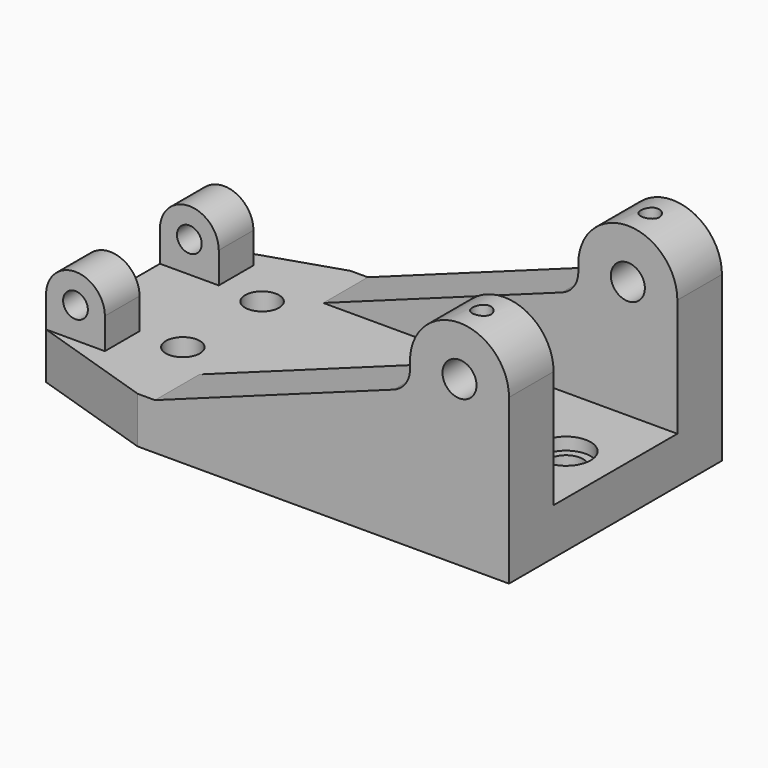
from build123d import *

# Parameters (mm, degrees)
F0_W            = 160
F0_H            = 86
F1_DEPTH        = 15
F3_DEPTH        = 18
F4_R            = 8
F6_D            = 11
F9_DEPTH        = 14
F11_D           = 8
F12_C1_SIZE2    = 13
F12_C1_SIZE     = 40
F12_C2_SIZE2    = 40
F12_C2_SIZE     = 13
F16_D           = 6
F16_DEPTH       = 12
F16_START       = 0.2837665
F16_TIP         = 1.8025818571
F18_D           = 11
F20_D           = 11
F20_CBORE_D     = 16
F20_CBORE_DEPTH = 4


# Not quite as in the source:
# - two fillets or chamfers of one size are made in one step
# - a pattern or mirror of a feature is missing from the dataset's text; its kind, count and spacing are read off the source's solid


with BuildPart() as f1:
    # F0 (on Top) → F1 (new body)
    with BuildSketch(Plane.XY):
        Rectangle(F0_W, F0_H)
    extrude(amount=F1_DEPTH)

    # F2 (on face) → F3 (join)
    with BuildSketch(Plane.XZ.offset(43)):
        with BuildLine():
            Line((48, 45), (-34.4243225836, 15))
            Line((-34.4243225836, 15), (80, 15))
            Line((80, 15), (80, 53))
            ThreePointArc((80, 53), (64, 69), (48, 53))
            Line((48, 53), (48, 45))
        make_face()
    f3 = extrude(amount=-F3_DEPTH)

    # F3_copies: F3 across plane
    add(f3.mirror(Plane.ZX))

    # F4
    f4_edges = [f1.edges().sort_by_distance(p)[0] for p in [
        (48, -34, 45),
        (48, 34, 45),
    ]]
    fillet(f4_edges, radius=F4_R)

    # F6 (through all)
    with Locations(Plane.XZ.offset(43)):
        with Locations((64, 53)):
            Hole(F6_D / 2)

    # F8 (on offset) → F9 (join)
    with BuildSketch(Plane.XZ.offset(30)):
        with BuildLine():
            Line((-80, 25), (-80, 15))
            Line((-80, 15), (-61, 15))
            Line((-61, 15), (-61, 25))
            ThreePointArc((-61, 25), (-70.5, 34.5), (-80, 25))
        make_face()
    f9 = extrude(amount=-F9_DEPTH)

    # F9_copies: F9 across plane
    add(f9.mirror(Plane.ZX))

    # F11 (through all)
    with Locations(Plane.XZ.offset(30)):
        with Locations((-70.5, 25)):
            Hole(F11_D / 2)

    # F12: chamfer of 40 x 13 on 2 edges, made by hand

    # F12_c1
    f12_c1_edges = [f1.edges().sort_by_distance(p)[0] for p in [
        (-80, -43, 7.5),
    ]]
    f12_c1_side = f1.faces().sort_by_distance((-79.74, -43, 7.5))[0]
    chamfer(f12_c1_edges, length=F12_C1_SIZE, length2=F12_C1_SIZE2, reference=f12_c1_side)

    # F12_c2
    f12_c2_edges = [f1.edges().sort_by_distance(p)[0] for p in [
        (-80, 43, 7.5),
    ]]
    f12_c2_side = f1.faces().sort_by_distance((-80, 42.74, 7.5))[0]
    chamfer(f12_c2_edges, length=F12_C2_SIZE, length2=F12_C2_SIZE2, reference=f12_c2_side)

    # F16
    # its depths count from where the whole tool has entered the part; down to there all is cleared
    with Locations(Plane.XY.offset(69).offset(-F16_START)):
        with Locations((64, -34), (64, 34)):
            Hole(F16_D / 2, depth=F16_DEPTH)
            with Locations((0, 0, -(F16_DEPTH + F16_TIP / 2))):  # 118° drill point
                Cone(0, F16_D / 2, F16_TIP, mode=Mode.SUBTRACT)

    # F18 (through all)
    with Locations(Plane.XY.offset(15)):
        with Locations((-47, -16), (-47, 16)):
            Hole(F18_D / 2)

    # F20 (through all)
    with Locations(Plane.XY.offset(15)):
        with Locations((64, 0)):
            CounterBoreHole(F20_D / 2, F20_CBORE_D / 2, F20_CBORE_DEPTH)


solid = f1.part
